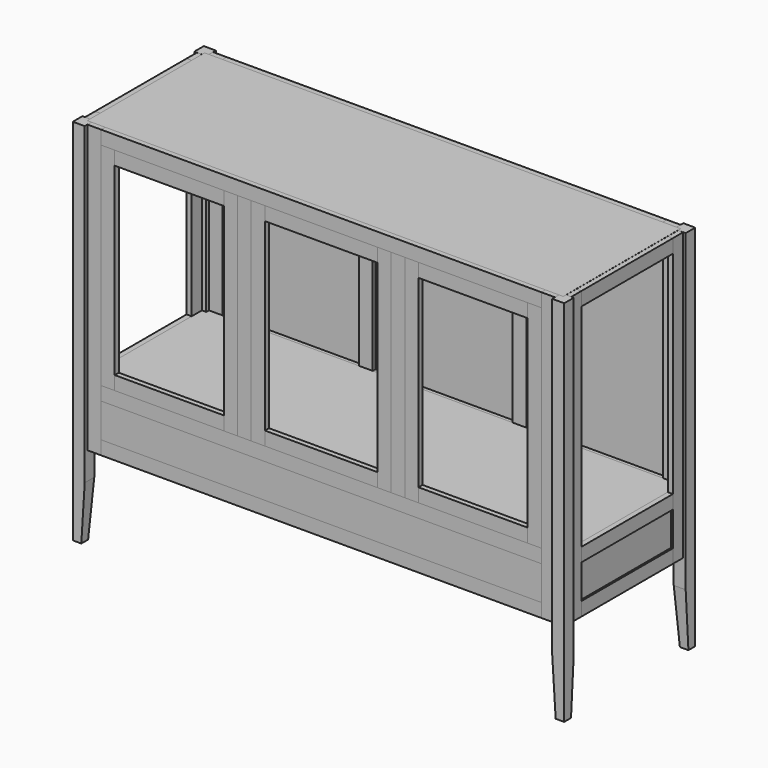
from build123d import *

# Parameters (mm, degrees)
F0_W      = 44.45
F0_H      = 1371.6
F1_DEPTH  = 44.45
F3_DEPTH  = 44.451
F5_DEPTH  = 44.451
F8_W      = 47.625
F8_H      = 1066.8
F9_DEPTH  = 19.05
F11_W     = 425.45
F11_H     = 50.8
F12_DEPTH = 19.05
F13_W     = 425.45
F13_H     = 50.8
F14_DEPTH = 19.05
F15_W     = 425.45
F15_H     = 50.8
F16_DEPTH = 19.05
F18_W     = 425.45
F18_H     = 127
F19_DEPTH = 6.35
F23_W     = 50.8
F23_H     = 1067.1170648575
F24_DEPTH = 19.05
F25_W     = 1638.3
F25_H     = 50.8
F26_DEPTH = 19.05
F28_W     = 1638.3
F28_H     = 50.8
F29_DEPTH = 19.05
F30_W     = 1638.3
F30_H     = 50.8
F31_DEPTH = 19.05
F32_W     = 50.8
F32_H     = 787.7170648575
F33_DEPTH = 19.05
F36_W     = 50.8
F36_H     = 787.7170648575
F37_DEPTH = 19.05
F38_W     = 50.8
F38_H     = 787.7170648575
F39_DEPTH = 19.05
F40_W     = 406.4
F40_H     = 50.8
F41_DEPTH = 19.05
F42_W     = 406.4
F42_H     = 50.8
F43_DEPTH = 19.05
F45_W     = 50.8
F45_H     = 787.7170648575
F46_DEPTH = 19.05
F47_W     = 50.8
F47_H     = 787.7170648575
F48_DEPTH = 19.05
F49_W     = 419.1
F49_H     = 50.8
F50_DEPTH = 19.05
F51_W     = 419.1
F51_H     = 50.8
F52_DEPTH = 19.05
F53_W     = 1771.65
F53_H     = 546.1
F54_DEPTH = 19.05
F55_W     = 1771.65
F55_H     = 546.1
F56_DEPTH = 19.05
F57_W     = 1638.3
F57_H     = 127
F58_DEPTH = 6.35
F59_W     = 1638.3
F59_H     = 127
F60_DEPTH = 25.4
F61_W     = 508
F61_H     = 787.7170648575
F62_DEPTH = 6.35
F61_W_2   = 520.7
F63_W     = 1771.65
F63_H     = 546.1
F64_DEPTH = 6.35


# Not quite as in the source:
# - a feature names something its author has since deleted; it is built from what else it names


with BuildPart() as f1:
    # F0 (on Front) → F1 (new body)
    with BuildSketch(Plane.XZ):
        with Locations((-606.7248311718, 685.8)):
            Rectangle(F0_W, F0_H)
    extrude(amount=F1_DEPTH)

    # F2 (on face) → F3 (cut, through all)
    with BuildSketch(Plane.XZ.offset(44.45)):
        Polygon((-584.4998311718, 203.2), (-597.1998311718, 0), (-584.4998311718, 0), align=None)
    extrude(amount=-F3_DEPTH, mode=Mode.SUBTRACT)

    # F4 (on face) → F5 (cut, through all)
    with BuildSketch(Plane(origin=(-628.9498311718, 0, 0), x_dir=(0, -1, 0), z_dir=(-1, 0, 0))):
        Polygon((12.7, 0), (0, 203.2), (0, 0), align=None)
    extrude(amount=-F5_DEPTH, mode=Mode.SUBTRACT)

    # F8 (on offset) → F9 (join)
    with BuildSketch(Plane(origin=(-619.4248311718, 0, 0), x_dir=(0, -1, 0), z_dir=(-1, 0, 0))):
        with Locations((-23.8125, 837.8829351425)):
            Rectangle(F8_W, F8_H)
    extrude(amount=-F9_DEPTH)


with BuildPart() as f10_1:
    # F10: instance of F1
    add(f1.part.mirror(Plane(origin=(-607.1138401808, 260.35, 699.1636036036), x_dir=(1, 0, 0), z_dir=(0, -1, 0))))


with BuildPart() as f12:
    # F11 (on offset) → F12 (new body)
    with BuildSketch(Plane(origin=(-619.4248311718, 0, 0), x_dir=(0, -1, 0), z_dir=(-1, 0, 0))):
        with Locations((-260.35, 1345.8829351425)):
            Rectangle(F11_W, F11_H)
    extrude(amount=-F12_DEPTH)


with BuildPart() as f14:
    # F13 (on offset) → F14 (new body)
    with BuildSketch(Plane(origin=(-619.4248311718, 0, 0), x_dir=(0, -1, 0), z_dir=(-1, 0, 0))):
        with Locations((-260.35, 329.8829351425)):
            Rectangle(F13_W, F13_H)
    extrude(amount=-F14_DEPTH)


with BuildPart() as f16:
    # F15 (on offset) → F16 (new body)
    with BuildSketch(Plane(origin=(-619.4248311718, 0, 0), x_dir=(0, -1, 0), z_dir=(-1, 0, 0))):
        with Locations((-260.35, 507.6829351425)):
            Rectangle(F15_W, F15_H)
    extrude(amount=-F16_DEPTH)


with BuildPart() as f19:
    # F18 (on offset) → F19 (new body)
    with BuildSketch(Plane(origin=(-613.0748311718, 0, 0), x_dir=(0, -1, 0), z_dir=(-1, 0, 0))):
        with Locations((-260.35, 418.7829351425)):
            Rectangle(F18_W, F18_H)
    extrude(amount=-F19_DEPTH)


with BuildPart() as f21_1:
    # F21: instance of F1
    add(f1.part.mirror(Plane(origin=(285.4501688282, -22.614009009, 699.1636036036), x_dir=(0, -1, 0), z_dir=(-1, 0, 0))))


with BuildPart() as f21_2:
    # F21: instance of F14
    add(f14.part.mirror(Plane(origin=(285.4501688282, -22.614009009, 699.1636036036), x_dir=(0, -1, 0), z_dir=(-1, 0, 0))))


with BuildPart() as f21_3:
    # F21: instance of F12
    add(f12.part.mirror(Plane(origin=(285.4501688282, -22.614009009, 699.1636036036), x_dir=(0, -1, 0), z_dir=(-1, 0, 0))))


with BuildPart() as f21_4:
    # F21: instance of F10_1
    add(f10_1.part.mirror(Plane(origin=(285.4501688282, -22.614009009, 699.1636036036), x_dir=(0, -1, 0), z_dir=(-1, 0, 0))))


with BuildPart() as f21_5:
    # F21: instance of F16
    add(f16.part.mirror(Plane(origin=(285.4501688282, -22.614009009, 699.1636036036), x_dir=(0, -1, 0), z_dir=(-1, 0, 0))))


with BuildPart() as f21_6:
    # F21: instance of F19
    add(f19.part.mirror(Plane(origin=(285.4501688282, -22.614009009, 699.1636036036), x_dir=(0, -1, 0), z_dir=(-1, 0, 0))))


with BuildPart() as f24:
    # F23 (on offset) → F24 (new body)
    with BuildSketch(Plane.XZ.offset(31.75)):
        with Locations((-559.0998311718, 838.0414675713)):
            Rectangle(F23_W, F23_H)
    extrude(amount=-F24_DEPTH)


with BuildPart() as f26:
    # F25 (on offset) → F26 (new body)
    with BuildSketch(Plane.XZ.offset(31.75)):
        with Locations((285.4501688282, 1346.2)):
            Rectangle(F25_W, F25_H)
    extrude(amount=-F26_DEPTH)


with BuildPart() as f27_1:
    # F27: instance of F24
    add(f24.part.mirror(Plane(origin=(285.4501688282, -22.614009009, 699.1636036036), x_dir=(0, -1, 0), z_dir=(-1, 0, 0))))


with BuildPart() as f29:
    # F28 (on offset) → F29 (new body)
    with BuildSketch(Plane.XZ.offset(31.75)):
        with Locations((285.4501688282, 329.8829351425)):
            Rectangle(F28_W, F28_H)
    extrude(amount=-F29_DEPTH)


with BuildPart() as f31:
    # F30 (on offset) → F31 (new body)
    with BuildSketch(Plane.XZ.offset(31.75)):
        with Locations((285.4501688282, 507.6829351425)):
            Rectangle(F30_W, F30_H)
    extrude(amount=-F31_DEPTH)


with BuildPart() as f33:
    # F32 (on offset) → F33 (new body)
    with BuildSketch(Plane.XZ.offset(31.75)):
        with Locations((-0.2998311718, 926.9414675713)):
            Rectangle(F32_W, F32_H)
    extrude(amount=-F33_DEPTH)


with BuildPart() as f34_1:
    # F34: instance of F33
    add(f33.part.mirror(Plane(origin=(285.4501688282, -22.614009009, 699.1636036036), x_dir=(0, -1, 0), z_dir=(-1, 0, 0))))


with BuildPart() as f35_1:
    # F35: instance of F24
    add(f24.part.mirror(Plane(origin=(-607.1138401808, 260.35, 699.1636036036), x_dir=(1, 0, 0), z_dir=(0, -1, 0))))


with BuildPart() as f35_2:
    # F35: instance of F26
    add(f26.part.mirror(Plane(origin=(-607.1138401808, 260.35, 699.1636036036), x_dir=(1, 0, 0), z_dir=(0, -1, 0))))


with BuildPart() as f35_3:
    # F35: instance of F33
    add(f33.part.mirror(Plane(origin=(-607.1138401808, 260.35, 699.1636036036), x_dir=(1, 0, 0), z_dir=(0, -1, 0))))


with BuildPart() as f35_4:
    # F35: instance of F34_1
    add(f34_1.part.mirror(Plane(origin=(-607.1138401808, 260.35, 699.1636036036), x_dir=(1, 0, 0), z_dir=(0, -1, 0))))


with BuildPart() as f35_5:
    # F35: instance of F27_1
    add(f27_1.part.mirror(Plane(origin=(-607.1138401808, 260.35, 699.1636036036), x_dir=(1, 0, 0), z_dir=(0, -1, 0))))


with BuildPart() as f35_6:
    # F35: instance of F31
    add(f31.part.mirror(Plane(origin=(-607.1138401808, 260.35, 699.1636036036), x_dir=(1, 0, 0), z_dir=(0, -1, 0))))


with BuildPart() as f35_7:
    # F35: instance of F29
    add(f29.part.mirror(Plane(origin=(-607.1138401808, 260.35, 699.1636036036), x_dir=(1, 0, 0), z_dir=(0, -1, 0))))


with BuildPart() as f37:
    # F36 (on offset) → F37 (new body)
    with BuildSketch(Plane.XZ.offset(31.75)):
        with Locations((-508.2998311718, 926.9414675713)):
            Rectangle(F36_W, F36_H)
    extrude(amount=-F37_DEPTH)


with BuildPart() as f39:
    # F38 (on offset) → F39 (new body)
    with BuildSketch(Plane.XZ.offset(31.75)):
        with Locations((-51.0998311718, 926.9414675713)):
            Rectangle(F38_W, F38_H)
    extrude(amount=-F39_DEPTH)


with BuildPart() as f41:
    # F40 (on offset) → F41 (new body)
    with BuildSketch(Plane.XZ.offset(31.75)):
        with Locations((-279.6998311718, 1295.4)):
            Rectangle(F40_W, F40_H)
    extrude(amount=-F41_DEPTH)


with BuildPart() as f43:
    # F42 (on offset) → F43 (new body)
    with BuildSketch(Plane.XZ.offset(31.75)):
        with Locations((-279.6998311718, 558.4829351425)):
            Rectangle(F42_W, F42_H)
    extrude(amount=-F43_DEPTH)


with BuildPart() as f44_1:
    # F44: instance of F37
    add(f37.part.mirror(Plane(origin=(285.4501688282, -22.614009009, 699.1636036036), x_dir=(0, -1, 0), z_dir=(-1, 0, 0))))


with BuildPart() as f44_2:
    # F44: instance of F41
    add(f41.part.mirror(Plane(origin=(285.4501688282, -22.614009009, 699.1636036036), x_dir=(0, -1, 0), z_dir=(-1, 0, 0))))


with BuildPart() as f44_3:
    # F44: instance of F39
    add(f39.part.mirror(Plane(origin=(285.4501688282, -22.614009009, 699.1636036036), x_dir=(0, -1, 0), z_dir=(-1, 0, 0))))


with BuildPart() as f44_4:
    # F44: instance of F43
    add(f43.part.mirror(Plane(origin=(285.4501688282, -22.614009009, 699.1636036036), x_dir=(0, -1, 0), z_dir=(-1, 0, 0))))


with BuildPart() as f46:
    # F45 (on offset) → F46 (new body)
    with BuildSketch(Plane.XZ.offset(31.75)):
        with Locations((50.5001688282, 926.9414675713)):
            Rectangle(F45_W, F45_H)
    extrude(amount=-F46_DEPTH)


with BuildPart() as f48:
    # F47 (on offset) → F48 (new body)
    with BuildSketch(Plane.XZ.offset(31.75)):
        with Locations((520.4001688282, 926.9414675713)):
            Rectangle(F47_W, F47_H)
    extrude(amount=-F48_DEPTH)


with BuildPart() as f50:
    # F49 (on offset) → F50 (new body)
    with BuildSketch(Plane.XZ.offset(31.75)):
        with Locations((285.4501688282, 1295.4)):
            Rectangle(F49_W, F49_H)
    extrude(amount=-F50_DEPTH)


with BuildPart() as f52:
    # F51 (on offset) → F52 (new body)
    with BuildSketch(Plane.XZ.offset(31.75)):
        with Locations((285.4501688282, 558.4829351425)):
            Rectangle(F51_W, F51_H)
    extrude(amount=-F52_DEPTH)


with BuildPart() as f54:
    # F53 (on face) → F54 (new body)
    with BuildSketch(Plane.XY.offset(1371.6)):
        with Locations((285.4501688282, 260.35)):
            Rectangle(F53_W, F53_H)
    extrude(amount=-F54_DEPTH)


with BuildPart() as f56:
    # F55 (on face) → F56 (new body)
    with BuildSketch(Plane(origin=(0, 0, 304.4829351425), x_dir=(1, 0, 0), z_dir=(0, 0, -1))):
        with Locations((285.4501688282, -260.35)):
            Rectangle(F55_W, F55_H)
    extrude(amount=-F56_DEPTH)


with BuildPart() as f58:
    # F57 (on face) → F58 (new body)
    with BuildSketch(Plane.XZ.offset(31.75)):
        with Locations((285.4501688282, 418.7829351425)):
            Rectangle(F57_W, F57_H)
    extrude(amount=-F58_DEPTH)


with BuildPart() as f60:
    # F59 (on face) → F60 (new body)
    with BuildSketch(Plane(origin=(0, 552.45, 0), x_dir=(-1, 0, 0), z_dir=(0, 1, 0))):
        with Locations((-285.4501688282, 418.7829351425)):
            Rectangle(F59_W, F59_H)
    extrude(amount=-F60_DEPTH)


with BuildPart() as f62:
    # F61 (on face) → F62 (new body)
    with BuildSketch(Plane(origin=(0, 552.45, 0), x_dir=(-1, 0, 0), z_dir=(0, 1, 0))):
        with Locations((-850.6001688282, 926.9414675713)):
            Rectangle(F61_W, F61_H)
    extrude(amount=-F62_DEPTH)


with BuildPart() as f62b:
    # F61 (on face) → F62, piece 2 (new body)
    with BuildSketch(Plane(origin=(0, 552.45, 0), x_dir=(-1, 0, 0), z_dir=(0, 1, 0))):
        with Locations((-285.4501688282, 926.9414675713)):
            Rectangle(F61_W_2, F61_H)
    extrude(amount=-F62_DEPTH)


with BuildPart() as f62c:
    # F61 (on face) → F62, piece 3 (new body)
    with BuildSketch(Plane(origin=(0, 552.45, 0), x_dir=(-1, 0, 0), z_dir=(0, 1, 0))):
        with Locations((279.6998311718, 926.9414675713)):
            Rectangle(F61_W, F61_H)
    extrude(amount=-F62_DEPTH)


with BuildPart() as f64:
    # F63 (on face) → F64 (new body)
    with BuildSketch(Plane.XY.offset(533.0829351425)):
        with Locations((285.4501688282, 260.35)):
            Rectangle(F63_W, F63_H)
    extrude(amount=-F64_DEPTH)


solid = Compound([f1.part, f10_1.part, f12.part, f14.part, f16.part, f19.part, f21_1.part, f21_2.part, f21_3.part, f21_4.part, f21_5.part, f21_6.part, f24.part, f26.part, f27_1.part, f29.part, f31.part, f33.part, f34_1.part, f35_1.part, f35_2.part, f35_3.part, f35_4.part, f35_5.part, f35_6.part, f35_7.part, f37.part, f39.part, f41.part, f43.part, f44_1.part, f44_2.part, f44_3.part, f44_4.part, f46.part, f48.part, f50.part, f52.part, f54.part, f56.part, f58.part, f60.part, f62.part, f62b.part, f62c.part, f64.part])
